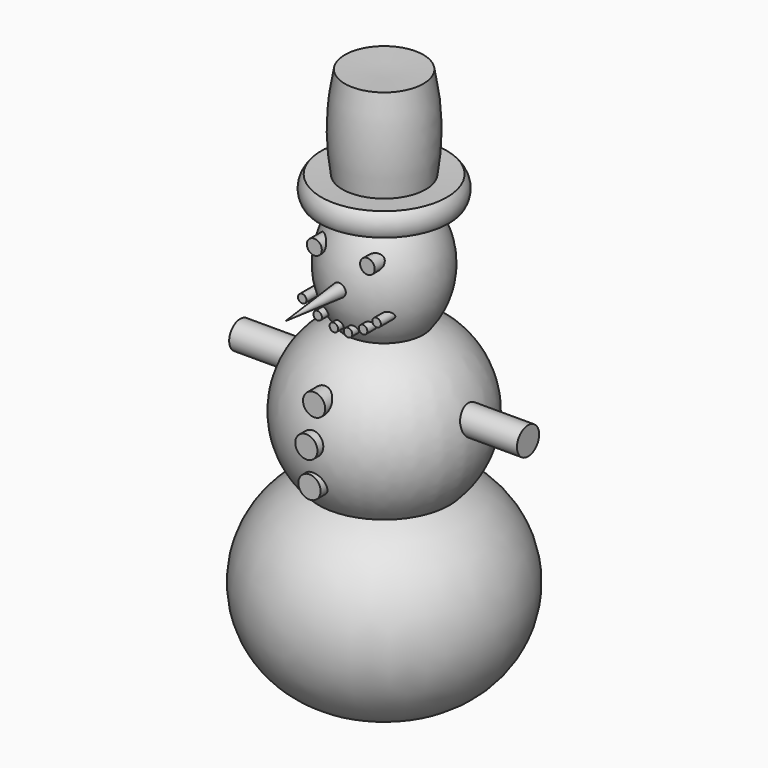
from build123d import *

# Parameters (mm, degrees)
F10_R     = 2.9031743956
F11_DEPTH = 22.86
F12_R     = 2.9031743956
F13_DEPTH = 25.4
F14_R     = 2.9031743956
F15_DEPTH = 24.384
F16_R     = 1.9156165745
F17_DEPTH = 13.716
F16_R_2   = 1.9517692667
F18_R     = 1.1044945862
F19_DEPTH = 14.224
F20_R     = 3.1058503017
F22_R     = 3.6123006976
F23_DEPTH = 37.592
F24_SCALE = 0.5


# Not quite as in the source:
# - an extrude whose draft closes it to a point is written as a loft to that point


with BuildPart() as f1:
    # F0 (on Front) → F1 (revolve)
    with BuildSketch(Plane.XZ):
        with BuildLine():
            Line((0, -37.033200264), (17.0688014477, -37.033200264))
            ThreePointArc((17.0688014477, -37.033200264), (23.4347196146, -16.7204253185), (10.260459967, 0))
            Line((10.260459967, 0), (0, 0))
            Line((0, 0), (0, -37.033200264))
        make_face()
    revolve(axis=Axis((0, 0, -18.516600132), (0, 0, -1)))


with BuildPart() as f3:
    # F2 (on Front) → F3 (revolve)
    with BuildSketch(Plane.XZ):
        with BuildLine():
            Line((0, -82.2097659111), (19.5554401726, -82.2097659111))
            ThreePointArc((19.5554401726, -82.2097659111), (32.0617990935, -58.5779997195), (16.649922356, -36.7298088968))
            Line((16.649922356, -36.7298088968), (0, -36.3972075284))
            Line((0, -36.3972075284), (0, -82.2097659111))
        make_face()
    revolve(axis=Axis((0, 0, -59.3034867197), (0, 0, -1)))


with BuildPart() as f5:
    # F4 (on Front) → F5 (revolve)
    with BuildSketch(Plane.XZ):
        with BuildLine():
            Line((0, 0), (10.2564934641, 0))
            ThreePointArc((10.2564934641, 0), (14.744146127, 14.0112577102), (9.0289367748, 27.5682024658))
            Line((9.0289367748, 27.5682024658), (0, 27.5682024658))
            Line((0, 27.5682024658), (0, 0))
        make_face()
    revolve(axis=Axis((0, 0, 13.7841012329), (0, 0, -1)))


with BuildPart() as f7:
    # F6 (on Front) → F7 (revolve)
    with BuildSketch(Plane.XZ):
        with BuildLine():
            Line((0, 27.777088806), (16.9282369316, 27.777088806))
            ThreePointArc((16.9282369316, 27.777088806), (17.6367783881, 30.7774312562), (16.4153152843, 33.6079989907))
            Line((16.4153152843, 33.6079989907), (0, 32.9180695117))
            Line((0, 32.9180695117), (0, 27.777088806))
        make_face()
    revolve(axis=Axis((0, 0, 30.3475791588), (0, 0, -1)))


with BuildPart() as f9:
    # F8 (on Front) → F9 (revolve)
    with BuildSketch(Plane.XZ):
        with BuildLine():
            Line((0, 33.6122661829), (10.8817331493, 33.6122661829))
            ThreePointArc((10.8817331493, 33.6122661829), (11.6948933703, 45.6851331029), (10.2538028732, 57.6992332935))
            Line((10.2538028732, 57.6992332935), (0, 57.3502294719))
            Line((0, 57.3502294719), (0, 33.6122661829))
        make_face()
    revolve(axis=Axis((0, 0, 45.4812478274), (0, 0, -1)))


with BuildPart() as f11:
    # F10 (on Front) → F11 (new body)
    with BuildSketch(Plane.XZ):
        with Locations((0, -10.1333223283)):
            Circle(F10_R)
    extrude(amount=F11_DEPTH)


with BuildPart() as f13:
    # F12 (on Front) → F13 (new body)
    with BuildSketch(Plane.XZ):
        with Locations((0, -18.8022069633)):
            Circle(F12_R)
    extrude(amount=F13_DEPTH)


with BuildPart() as f15:
    # F14 (on Front) → F15 (new body)
    with BuildSketch(Plane.XZ):
        with Locations((0, -28.4480024129)):
            Circle(F14_R)
    extrude(amount=F15_DEPTH)


with BuildPart() as f17:
    # F16 (on Front) → F17 (new body)
    with BuildSketch(Plane.XZ):
        with Locations((6.5965889953, 20.0959835202)):
            Circle(F16_R)
    extrude(amount=F17_DEPTH)


with BuildPart() as f17b:
    # F16 (on Front) → F17, piece 2 (new body)
    with BuildSketch(Plane.XZ):
        with Locations((-7.2662262246, 20.0220234692)):
            Circle(F16_R_2)
    extrude(amount=F17_DEPTH)


with BuildPart() as f19:
    # F18 (on Front) → F19 (new body)
    with BuildSketch(Plane.XZ):
        with Locations((-10.0144315511, 7.4778371491)):
            Circle(F18_R)
    extrude(amount=F19_DEPTH)


with BuildPart() as f19b:
    # F18 (on Front) → F19, piece 2 (new body)
    with BuildSketch(Plane.XZ):
        with Locations((-5.9856851585, 4.8683495261)):
            Circle(F18_R)
    extrude(amount=F19_DEPTH)


with BuildPart() as f19c:
    # F18 (on Front) → F19, piece 3 (new body)
    with BuildSketch(Plane.XZ):
        with Locations((-1.765095978, 3.535436932)):
            Circle(F18_R)
    extrude(amount=F19_DEPTH)


with BuildPart() as f19d:
    # F18 (on Front) → F19, piece 4 (new body)
    with BuildSketch(Plane.XZ):
        with Locations((1.9503422081, 3.5495357588)):
            Circle(F18_R)
    extrude(amount=F19_DEPTH)


with BuildPart() as f19e:
    # F18 (on Front) → F19, piece 5 (new body)
    with BuildSketch(Plane.XZ):
        with Locations((9.4110434875, 8.2946131006)):
            Circle(F18_R)
    extrude(amount=F19_DEPTH)


with BuildPart() as f19f:
    # F18 (on Front) → F19, piece 6 (new body)
    with BuildSketch(Plane.XZ):
        with Locations((5.8838534169, 5.5207260884)):
            Circle(F18_R)
    extrude(amount=F19_DEPTH)


with BuildPart() as f21:
    # F20 (on Front) → F21 section 0
    with BuildSketch(Plane.XZ, mode=Mode.PRIVATE) as f21_s0:
        with Locations((0, 12.8816543147)):
            Circle(F20_R)
    loft([f21_s0.sketch, Vertex(0, -32.2554886542, 12.8816543147)], ruled=True)


with BuildPart() as f23:
    # F22 (on Right) → F23 (new body, symmetric)
    with BuildSketch(Plane.YZ):
        with Locations((0, -15.5192539096)):
            Circle(F22_R)
    extrude(amount=F23_DEPTH, both=True)


with BuildPart() as f17b_1:
    # F24: moved
    add(f17b.part.scale(F24_SCALE))


with BuildPart() as f19_1:
    # F24: moved
    add(f19.part.scale(F24_SCALE))


with BuildPart() as f19b_1:
    # F24: moved
    add(f19b.part.scale(F24_SCALE))


with BuildPart() as f19e_1:
    # F24: moved
    add(f19e.part.scale(F24_SCALE))


with BuildPart() as f19f_1:
    # F24: moved
    add(f19f.part.scale(F24_SCALE))


with BuildPart() as f1_1:
    # F24: moved
    add(f1.part.scale(F24_SCALE))


with BuildPart() as f3_1:
    # F24: moved
    add(f3.part.scale(F24_SCALE))


with BuildPart() as f5_1:
    # F24: moved
    add(f5.part.scale(F24_SCALE))


with BuildPart() as f7_1:
    # F24: moved
    add(f7.part.scale(F24_SCALE))


with BuildPart() as f9_1:
    # F24: moved
    add(f9.part.scale(F24_SCALE))


with BuildPart() as f11_1:
    # F24: moved
    add(f11.part.scale(F24_SCALE))


with BuildPart() as f13_1:
    # F24: moved
    add(f13.part.scale(F24_SCALE))


with BuildPart() as f15_1:
    # F24: moved
    add(f15.part.scale(F24_SCALE))


with BuildPart() as f17_1:
    # F24: moved
    add(f17.part.scale(F24_SCALE))


with BuildPart() as f23_1:
    # F24: moved
    add(f23.part.scale(F24_SCALE))


with BuildPart() as f19c_1:
    # F24: moved
    add(f19c.part.scale(F24_SCALE))


with BuildPart() as f19d_1:
    # F24: moved
    add(f19d.part.scale(F24_SCALE))


with BuildPart() as f21_1:
    # F24: moved
    add(f21.part.scale(F24_SCALE))


solid = Compound([f17b_1.part, f19_1.part, f19b_1.part, f19e_1.part, f19f_1.part, f1_1.part, f3_1.part, f5_1.part, f7_1.part, f9_1.part, f11_1.part, f13_1.part, f15_1.part, f17_1.part, f23_1.part, f19c_1.part, f19d_1.part, f21_1.part])
